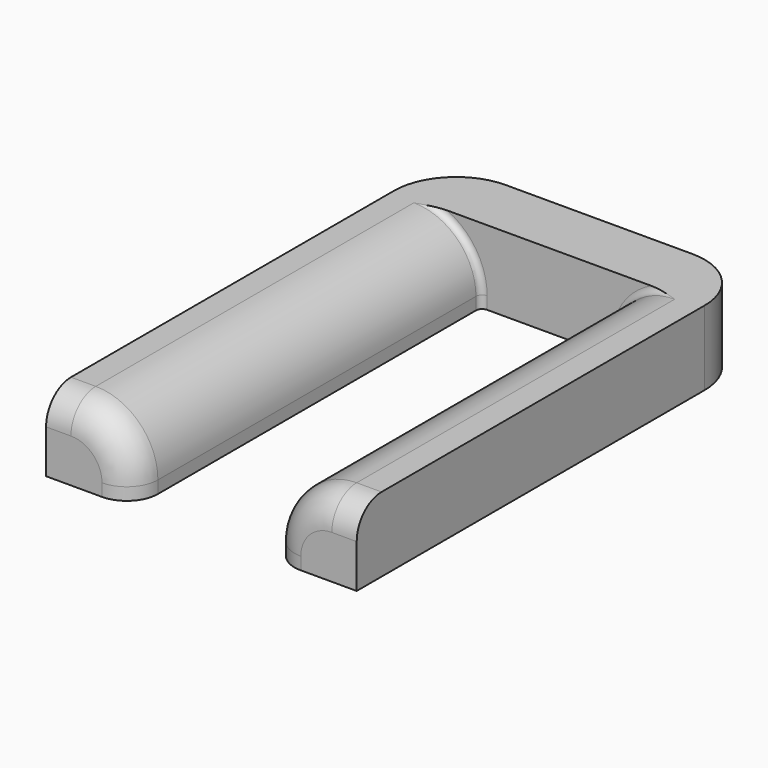
from build123d import *

# Parameters (mm, degrees)
F0_W         = 50
F0_H         = 12
F1_DEPTH     = 10
F2_W         = 14
F2_H         = 12
F3_DEPTH     = 70
F4_R         = 10
F5_R         = 5
F6_T1_DEPTH  = 2
F6_T6_ANGLE  = 132.9890967712
F6_T12_ANGLE = 132.9890967712
F7_R         = 10


# Not quite as in the source:
# - a fillet or chamfer that OpenCascade refuses, or shapes differently, is made with other operations: its cross-section is extruded or revolved along the edge and cut away or added


with BuildPart() as f1:
    # F0 (on Front) → F1 (new body)
    with BuildSketch(Plane.XZ):
        with Locations((25, 6)):
            Rectangle(F0_W, F0_H)
    extrude(amount=F1_DEPTH)

    # F2 (on face) → F3 (join)
    with BuildSketch(Plane.XZ.offset(10)):
        with Locations((7, 6)):
            Rectangle(F2_W, F2_H)
        with Locations((43, 6)):
            Rectangle(F2_W, F2_H)
    extrude(amount=F3_DEPTH)

    # F4
    f4_edges = [f1.edges().sort_by_distance(p)[0] for p in [
        (14, -45, 12),
        (36, -45, 12),
    ]]
    fillet(f4_edges, radius=F4_R)

    # F5
    f5_edges = [f1.edges().sort_by_distance(p)[0] for p in [
        (11.071068, -80, 9.071068),
        (38.928932, -80, 9.071068),
        (48, -80, 12),
        (36, -80, 1),
        (2, -80, 12),
        (14, -80, 1),
    ]]
    fillet(f5_edges, radius=F5_R)

    # F6: fillet of radius 1 on 4 edges, made by hand

    # F6_s2 → F6_t1 (join)
    with BuildSketch(Plane.XY):
        with BuildLine():
            ThreePointArc((14, -11), (14.2928932188, -10.2928932188), (15, -10))
            Line((15, -10), (14, -10))
            Line((14, -10), (14, -11))
        make_face()
        with BuildLine():
            ThreePointArc((35, -10), (35.7071067812, -10.2928932188), (36, -11))
            Line((36, -11), (36, -10))
            Line((36, -10), (35, -10))
        make_face()
    extrude(amount=F6_T1_DEPTH)


with BuildPart() as f6_tool4:
    # F6_s5 → F6_t6 (revolve)
    with BuildSketch(Plane.XY.offset(2)):
        with BuildLine():
            ThreePointArc((15, -10), (14.2928932188, -10.2928932188), (14, -11))
            Line((14, -11), (14, -10))
            Line((14, -10), (15, -10))
        make_face()
    revolve(axis=Axis((4, -10, 2), (0, -1, 0)), revolution_arc=F6_T6_ANGLE)

    split(bisect_by=Plane.XY.offset(12), keep=Keep.BOTTOM)

    split(bisect_by=Plane.YZ, keep=Keep.TOP)


with BuildPart() as f1_1:
    add(f1.part)

    # F6_t3: union F6_tool4
    add(f6_tool4.part)


with BuildPart() as f6_tool10:
    # F6_s11 → F6_t12 (revolve)
    with BuildSketch(Plane.XY.offset(2)):
        with BuildLine():
            ThreePointArc((35, -10), (35.7071067812, -10.2928932188), (36, -11))
            Line((36, -11), (36, -10))
            Line((36, -10), (35, -10))
        make_face()
    revolve(axis=Axis((46, -10, 2), (0, 1, 0)), revolution_arc=F6_T12_ANGLE)

    split(bisect_by=Plane.YZ.offset(50), keep=Keep.BOTTOM)

    split(bisect_by=Plane.XY.offset(12), keep=Keep.BOTTOM)


with BuildPart() as f1_2:
    add(f1_1.part)

    # F6_t9: union F6_tool10
    add(f6_tool10.part)

    # F7
    f7_edges = [f1_2.edges().sort_by_distance(p)[0] for p in [
        (50, 0, 6),
        (0, 0, 6),
    ]]
    fillet(f7_edges, radius=F7_R)


solid = f1_2.part
